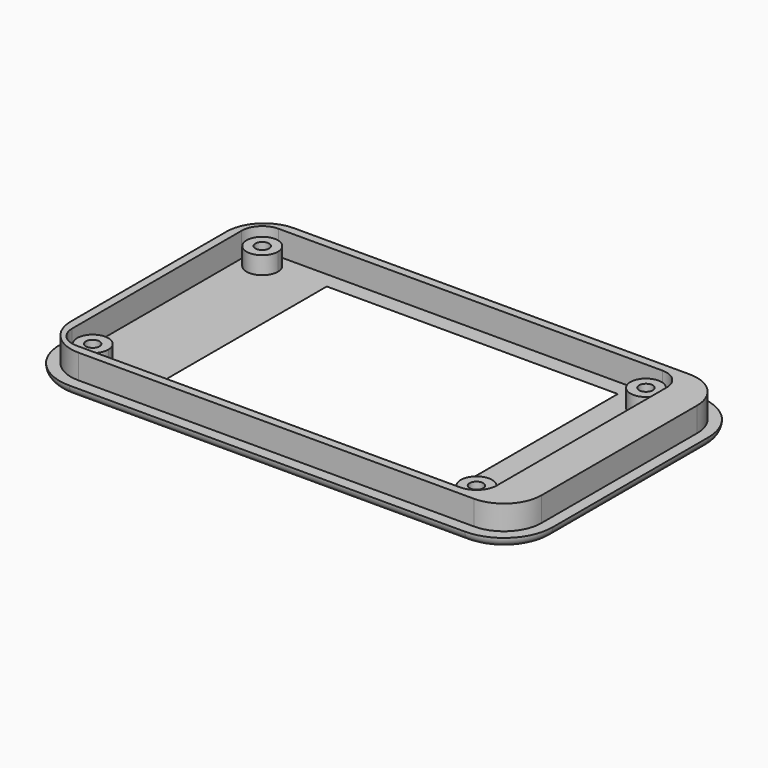
from build123d import *

# Parameters (mm, degrees)
F1_DEPTH = 5.6
F2_DEPTH = 7
F0_W     = 59.6
F0_H     = 45.2
F3_DEPTH = 2
F4_R     = 1.99999
F5_SIZE2 = 1.99999
F5_SIZE  = 2.99999
F6_R     = 1.4
F7_DEPTH = 5


# Not quite as in the source:
# - a fillet or chamfer is up to 0.001 mm smaller than in the source, because OpenCascade refuses the exact size


with BuildPart() as f1:
    # F0 (on Top) → F1 (new body)
    with BuildSketch(Plane.XY):
        with BuildLine():
            ThreePointArc((-34.4414402544, 28.5581715763), (-31.2414402544, 25.3581715763), (-28.0414402544, 28.5581715763))
            ThreePointArc((-28.0414402544, 28.5581715763), (-28.9786985547, 30.8209132761), (-31.2414402544, 31.7581715763))
            ThreePointArc((-31.2414402544, 31.7581715763), (-33.5041819542, 30.8209132761), (-34.4414402544, 28.5581715763))
        make_face()
    extrude(amount=F1_DEPTH)



with BuildPart() as f1b:
    # F0 (on Top) → F1, piece 2 (new body)
    with BuildSketch(Plane.XY):
        with BuildLine():
            ThreePointArc((-28.0414402544, -14.8418284237), (-31.2414402544, -11.6418284237), (-34.4414402544, -14.8418284237))
            ThreePointArc((-34.4414402544, -14.8418284237), (-33.5041819542, -17.1045701235), (-31.2414402544, -18.0418284237))
            ThreePointArc((-31.2414402544, -18.0418284237), (-28.9786985547, -17.1045701235), (-28.0414402544, -14.8418284237))
        make_face()
    extrude(amount=F1_DEPTH)


with BuildPart() as f1c:
    # F0 (on Top) → F1, piece 3 (new body)
    with BuildSketch(Plane.XY):
        with BuildLine():
            ThreePointArc((47.3585597456, -18.0418284237), (49.6213014453, -17.1045701235), (50.5585597456, -14.8418284237))
            ThreePointArc((50.5585597456, -14.8418284237), (45.0958180458, -12.5790867239), (47.3585597456, -18.0418284237))
        make_face()
    extrude(amount=F1_DEPTH)


with BuildPart() as f1d:
    # F0 (on Top) → F1, piece 4 (new body)
    with BuildSketch(Plane.XY):
        with BuildLine():
            ThreePointArc((50.5585597456, 28.5581715763), (49.6213014453, 30.8209132761), (47.3585597456, 31.7581715763))
            ThreePointArc((47.3585597456, 31.7581715763), (45.0958180458, 26.2954298765), (50.5585597456, 28.5581715763))
        make_face()
    extrude(amount=F1_DEPTH)


with BuildPart() as f2:
    # F0 (on Top) → F2 (new body)
    with BuildSketch(Plane.XY):
        with BuildLine():
            Line((51.5585597456, 34.4581715763), (-29.4414402544, 34.4581715763))
            ThreePointArc((-29.4414402544, 34.4581715763), (-34.8861624696, 32.2028937914), (-37.1414402544, 26.7581715763))
            Line((-37.1414402544, 26.7581715763), (-37.1414402544, -13.0418284237))
            ThreePointArc((-37.1414402544, -13.0418284237), (-34.8861624696, -18.4865506389), (-29.4414402544, -20.7418284237))
            Line((-29.4414402544, -20.7418284237), (51.5585597456, -20.7418284237))
            ThreePointArc((51.5585597456, -20.7418284237), (57.0032819607, -18.4865506389), (59.2585597456, -13.0418284237))
            Line((59.2585597456, -13.0418284237), (59.2585597456, 26.7581715763))
            ThreePointArc((59.2585597456, 26.7581715763), (57.0032819607, 32.2028937914), (51.5585597456, 34.4581715763))
        make_face()
        with BuildLine():
            ThreePointArc((47.3585597456, 32.7581715763), (50.3284082265, 31.5280200572), (51.5585597456, 28.5581715763))
            Line((51.5585597456, 28.5581715763), (51.5585597456, -14.8418284237))
            ThreePointArc((51.5585597456, -14.8418284237), (50.3284082265, -17.8116769047), (47.3585597456, -19.0418284237))
            Line((47.3585597456, -19.0418284237), (-31.2414402544, -19.0418284237))
            ThreePointArc((-31.2414402544, -19.0418284237), (-34.2112887354, -17.8116769047), (-35.4414402544, -14.8418284237))
            Line((-35.4414402544, -14.8418284237), (-35.4414402544, 28.5581715763))
            ThreePointArc((-35.4414402544, 28.5581715763), (-34.2112887354, 31.5280200572), (-31.2414402544, 32.7581715763))
            Line((-31.2414402544, 32.7581715763), (47.3585597456, 32.7581715763))
        make_face(mode=Mode.SUBTRACT)
    extrude(amount=F2_DEPTH)


with BuildPart() as f1_1:
    add(f1.part)

    add(f1b.part)  # F3 merges F1b

    add(f1c.part)  # F3 merges F1c

    add(f1d.part)  # F3 merges F1d

    add(f2.part)  # F3 merges F2
    # F0 (on Top) → F3 (join)
    with BuildSketch(Plane.XY):
        with BuildLine():
            Line((51.5585597456, 36.7581715763), (-29.4414402544, 36.7581715763))
            ThreePointArc((-29.4414402544, 36.7581715763), (-36.5125080663, 33.8292393881), (-39.4414402544, 26.7581715763))
            Line((-39.4414402544, 26.7581715763), (-39.4414402544, -13.0418284237))
            ThreePointArc((-39.4414402544, -13.0418284237), (-36.5125080663, -20.1128962356), (-29.4414402544, -23.0418284237))
            Line((-29.4414402544, -23.0418284237), (51.5585597456, -23.0418284237))
            ThreePointArc((51.5585597456, -23.0418284237), (58.6296275574, -20.1128962356), (61.5585597456, -13.0418284237))
            Line((61.5585597456, -13.0418284237), (61.5585597456, 26.7581715763))
            ThreePointArc((61.5585597456, 26.7581715763), (58.6296275574, 33.8292393881), (51.5585597456, 36.7581715763))
        make_face()
        with BuildLine():
            ThreePointArc((-37.1414402544, 26.7581715763), (-34.8861624696, 32.2028937914), (-29.4414402544, 34.4581715763))
            Line((-29.4414402544, 34.4581715763), (51.5585597456, 34.4581715763))
            ThreePointArc((51.5585597456, 34.4581715763), (57.0032819607, 32.2028937914), (59.2585597456, 26.7581715763))
            Line((59.2585597456, 26.7581715763), (59.2585597456, -13.0418284237))
            ThreePointArc((59.2585597456, -13.0418284237), (57.0032819607, -18.4865506389), (51.5585597456, -20.7418284237))
            Line((51.5585597456, -20.7418284237), (-29.4414402544, -20.7418284237))
            ThreePointArc((-29.4414402544, -20.7418284237), (-34.8861624696, -18.4865506389), (-37.1414402544, -13.0418284237))
            Line((-37.1414402544, -13.0418284237), (-37.1414402544, 26.7581715763))
        make_face(mode=Mode.SUBTRACT)
        with BuildLine():
            Line((51.5585597456, -14.8418284237), (51.5585597456, 28.5581715763))
            ThreePointArc((51.5585597456, 28.5581715763), (50.3284082265, 31.5280200572), (47.3585597456, 32.7581715763))
            Line((47.3585597456, 32.7581715763), (-31.2414402544, 32.7581715763))
            ThreePointArc((-31.2414402544, 32.7581715763), (-34.2112887354, 31.5280200572), (-35.4414402544, 28.5581715763))
            Line((-35.4414402544, 28.5581715763), (-35.4414402544, -14.8418284237))
            ThreePointArc((-35.4414402544, -14.8418284237), (-34.2112887354, -17.8116769047), (-31.2414402544, -19.0418284237))
            Line((-31.2414402544, -19.0418284237), (47.3585597456, -19.0418284237))
            ThreePointArc((47.3585597456, -19.0418284237), (50.3284082265, -17.8116769047), (51.5585597456, -14.8418284237))
        make_face()
        with BuildLine():
            ThreePointArc((-34.4414402544, 28.5581715763), (-33.5041819542, 30.8209132761), (-31.2414402544, 31.7581715763))
            Line((-31.2414402544, 31.7581715763), (47.3585597456, 31.7581715763))
            ThreePointArc((47.3585597456, 31.7581715763), (49.6213014453, 30.8209132761), (50.5585597456, 28.5581715763))
            Line((50.5585597456, 28.5581715763), (50.5585597456, -14.8418284237))
            ThreePointArc((50.5585597456, -14.8418284237), (49.6213014453, -17.1045701235), (47.3585597456, -18.0418284237))
            Line((47.3585597456, -18.0418284237), (-31.2414402544, -18.0418284237))
            ThreePointArc((-31.2414402544, -18.0418284237), (-33.5041819542, -17.1045701235), (-34.4414402544, -14.8418284237))
            Line((-34.4414402544, -14.8418284237), (-34.4414402544, 28.5581715763))
        make_face(mode=Mode.SUBTRACT)
        with BuildLine():
            ThreePointArc((-31.2414402544, 31.7581715763), (-28.9786985547, 30.8209132761), (-28.0414402544, 28.5581715763))
            ThreePointArc((-28.0414402544, 28.5581715763), (-31.2414402544, 25.3581715763), (-34.4414402544, 28.5581715763))
            Line((-34.4414402544, 28.5581715763), (-34.4414402544, -14.8418284237))
            ThreePointArc((-34.4414402544, -14.8418284237), (-31.2414402544, -11.6418284237), (-28.0414402544, -14.8418284237))
            ThreePointArc((-28.0414402544, -14.8418284237), (-28.9786985547, -17.1045701235), (-31.2414402544, -18.0418284237))
            Line((-31.2414402544, -18.0418284237), (47.3585597456, -18.0418284237))
            ThreePointArc((47.3585597456, -18.0418284237), (45.0958180458, -12.5790867239), (50.5585597456, -14.8418284237))
            Line((50.5585597456, -14.8418284237), (50.5585597456, 28.5581715763))
            ThreePointArc((50.5585597456, 28.5581715763), (45.0958180458, 26.2954298765), (47.3585597456, 31.7581715763))
            Line((47.3585597456, 31.7581715763), (-31.2414402544, 31.7581715763))
        make_face()
        with Locations((11.0585597456, 6.8581715763)):
            Rectangle(F0_W, F0_H, mode=Mode.SUBTRACT)
    extrude(amount=F3_DEPTH)

    # F4 (radius 2 in the source; OpenCascade refuses exactly that, so slightly less here)
    f4_edges = [f1_1.edges().sort_by_distance(p)[0] for p in [
        (-36.512508, -20.112896, 0),
    ]]
    fillet(f4_edges, radius=F4_R)

    # F5 (size 3 and 2 in the source; OpenCascade refuses exactly that, so slightly less here)
    f5_edges = [f1_1.edges().sort_by_distance(p)[0] for p in [
        (11.05856, 29.458172, 0),
        (-18.74144, 6.858172, 0),
        (11.05856, -15.741828, 0),
        (40.85856, 6.858172, 0),
    ]]
    f5_side = f1_1.faces().sort_by_distance((-34.307016, -17.907405, 0))[0]
    chamfer(f5_edges, length=F5_SIZE, length2=F5_SIZE2, reference=f5_side)

    # F6 (on face) → F7 (cut)
    with BuildSketch(Plane.XY.offset(5.6)):
        with Locations((-31.2414402544, 28.5581715763)):
            Circle(F6_R)
        with Locations((-31.2414402544, -14.8418284237)):
            Circle(F6_R)
        with Locations((47.3585597456, -14.8418284237)):
            Circle(F6_R)
        with Locations((47.3585597456, 28.5581715763)):
            Circle(F6_R)
    extrude(amount=-F7_DEPTH, mode=Mode.SUBTRACT)


solid = f1_1.part
